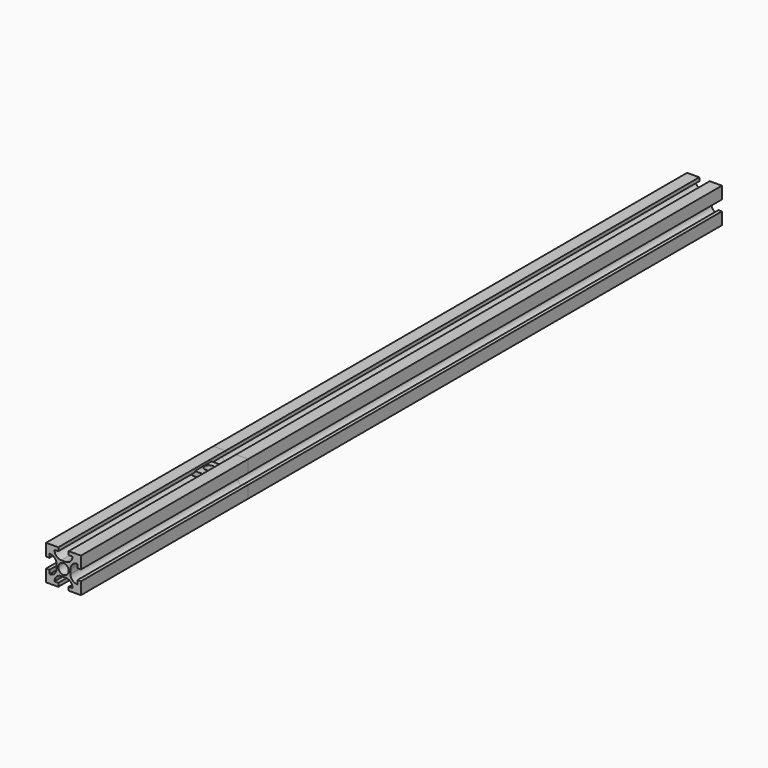
from build123d import *

# Parameters (mm, degrees)
F0_R      = 3
F1_DEPTH  = 350
F2_DEPTH  = 260
F3_DEPTH  = 460
F4_DEPTH  = 280
F5_DEPTH  = 210
F6_R      = 3
F7_DEPTH  = 20.001
F8_DEPTH  = 250
F10_DEPTH = 12
F11_R     = 2.5
F12_DEPTH = 18.701799197
F13_DEPTH = 460
F14_DEPTH = 227
F15_DEPTH = 340


with BuildPart() as f1:
    # F0 (on Front) → F1 (new body)
    with BuildSketch(Plane.XZ):
        with BuildLine():
            Line((3, 10), (3, 8))
            Line((3, 8), (5.1872519999, 8))
            ThreePointArc((5.1872519999, 8), (4.0330427178, 5.1732112188), (1.2140873587, 4))
            Line((1.2140873587, 4), (0, 4))
            Line((0, 4), (-1.2140873587, 4))
            ThreePointArc((-1.2140873587, 4), (-4.0330427178, 5.1732112188), (-5.1872519999, 8))
            Line((-5.1872519999, 8), (-3, 8))
            Line((-3, 8), (-3, 10))
            Line((-3, 10), (-10, 10))
            Line((-10, 10), (-10, 3))
            Line((-10, 3), (-8, 3))
            Line((-8, 3), (-8, 5.1872519999))
            ThreePointArc((-8, 5.1872519999), (-5.1732112188, 4.0330427178), (-4, 1.2140873587))
            Line((-4, 1.2140873587), (-4, 0))
            Line((-4, 0), (-4, -1.2140873587))
            ThreePointArc((-4, -1.2140873587), (-5.1732112188, -4.0330427178), (-8, -5.1872519999))
            Line((-8, -5.1872519999), (-8, -3))
            Line((-8, -3), (-10, -3))
            Line((-10, -3), (-10, -10))
            Line((-10, -10), (-3, -10))
            Line((-3, -10), (-3, -8))
            Line((-3, -8), (-5.1872519999, -8))
            ThreePointArc((-5.1872519999, -8), (-4.0330427178, -5.1732112188), (-1.2140873587, -4))
            Line((-1.2140873587, -4), (0, -4))
            Line((0, -4), (1.2140873587, -4))
            ThreePointArc((1.2140873587, -4), (4.0330427178, -5.1732112188), (5.1872519999, -8))
            Line((5.1872519999, -8), (3, -8))
            Line((3, -8), (3, -10))
            Line((3, -10), (10, -10))
            Line((10, -10), (10, -3))
            Line((10, -3), (8, -3))
            Line((8, -3), (8, -5.1872519999))
            ThreePointArc((8, -5.1872519999), (5.1732112188, -4.0330427178), (4, -1.2140873587))
            Line((4, -1.2140873587), (4, 0))
            Line((4, 0), (4, 1.2140873587))
            ThreePointArc((4, 1.2140873587), (5.1732112188, 4.0330427178), (8, 5.1872519999))
            Line((8, 5.1872519999), (8, 3))
            Line((8, 3), (10, 3))
            Line((10, 3), (10, 10))
            Line((10, 10), (3, 10))
        make_face()
        Circle(F0_R, mode=Mode.SUBTRACT)
    extrude(amount=F1_DEPTH)


with BuildPart() as f2:
    # F0 (on Front) → F2 (new body)
    with BuildSketch(Plane.XZ):
        with BuildLine():
            Line((3, 10), (3, 8))
            Line((3, 8), (5.1872519999, 8))
            ThreePointArc((5.1872519999, 8), (4.0330427178, 5.1732112188), (1.2140873587, 4))
            Line((1.2140873587, 4), (0, 4))
            Line((0, 4), (-1.2140873587, 4))
            ThreePointArc((-1.2140873587, 4), (-4.0330427178, 5.1732112188), (-5.1872519999, 8))
            Line((-5.1872519999, 8), (-3, 8))
            Line((-3, 8), (-3, 10))
            Line((-3, 10), (-10, 10))
            Line((-10, 10), (-10, 3))
            Line((-10, 3), (-8, 3))
            Line((-8, 3), (-8, 5.1872519999))
            ThreePointArc((-8, 5.1872519999), (-5.1732112188, 4.0330427178), (-4, 1.2140873587))
            Line((-4, 1.2140873587), (-4, 0))
            Line((-4, 0), (-4, -1.2140873587))
            ThreePointArc((-4, -1.2140873587), (-5.1732112188, -4.0330427178), (-8, -5.1872519999))
            Line((-8, -5.1872519999), (-8, -3))
            Line((-8, -3), (-10, -3))
            Line((-10, -3), (-10, -10))
            Line((-10, -10), (-3, -10))
            Line((-3, -10), (-3, -8))
            Line((-3, -8), (-5.1872519999, -8))
            ThreePointArc((-5.1872519999, -8), (-4.0330427178, -5.1732112188), (-1.2140873587, -4))
            Line((-1.2140873587, -4), (0, -4))
            Line((0, -4), (1.2140873587, -4))
            ThreePointArc((1.2140873587, -4), (4.0330427178, -5.1732112188), (5.1872519999, -8))
            Line((5.1872519999, -8), (3, -8))
            Line((3, -8), (3, -10))
            Line((3, -10), (10, -10))
            Line((10, -10), (10, -3))
            Line((10, -3), (8, -3))
            Line((8, -3), (8, -5.1872519999))
            ThreePointArc((8, -5.1872519999), (5.1732112188, -4.0330427178), (4, -1.2140873587))
            Line((4, -1.2140873587), (4, 0))
            Line((4, 0), (4, 1.2140873587))
            ThreePointArc((4, 1.2140873587), (5.1732112188, 4.0330427178), (8, 5.1872519999))
            Line((8, 5.1872519999), (8, 3))
            Line((8, 3), (10, 3))
            Line((10, 3), (10, 10))
            Line((10, 10), (3, 10))
        make_face()
        Circle(F0_R, mode=Mode.SUBTRACT)
    extrude(amount=F2_DEPTH)


with BuildPart() as f3:
    # F0 (on Front) → F3 (new body)
    with BuildSketch(Plane.XZ):
        with BuildLine():
            Line((3, 10), (3, 8))
            Line((3, 8), (5.1872519999, 8))
            ThreePointArc((5.1872519999, 8), (4.0330427178, 5.1732112188), (1.2140873587, 4))
            Line((1.2140873587, 4), (0, 4))
            Line((0, 4), (-1.2140873587, 4))
            ThreePointArc((-1.2140873587, 4), (-4.0330427178, 5.1732112188), (-5.1872519999, 8))
            Line((-5.1872519999, 8), (-3, 8))
            Line((-3, 8), (-3, 10))
            Line((-3, 10), (-10, 10))
            Line((-10, 10), (-10, 3))
            Line((-10, 3), (-8, 3))
            Line((-8, 3), (-8, 5.1872519999))
            ThreePointArc((-8, 5.1872519999), (-5.1732112188, 4.0330427178), (-4, 1.2140873587))
            Line((-4, 1.2140873587), (-4, 0))
            Line((-4, 0), (-4, -1.2140873587))
            ThreePointArc((-4, -1.2140873587), (-5.1732112188, -4.0330427178), (-8, -5.1872519999))
            Line((-8, -5.1872519999), (-8, -3))
            Line((-8, -3), (-10, -3))
            Line((-10, -3), (-10, -10))
            Line((-10, -10), (-3, -10))
            Line((-3, -10), (-3, -8))
            Line((-3, -8), (-5.1872519999, -8))
            ThreePointArc((-5.1872519999, -8), (-4.0330427178, -5.1732112188), (-1.2140873587, -4))
            Line((-1.2140873587, -4), (0, -4))
            Line((0, -4), (1.2140873587, -4))
            ThreePointArc((1.2140873587, -4), (4.0330427178, -5.1732112188), (5.1872519999, -8))
            Line((5.1872519999, -8), (3, -8))
            Line((3, -8), (3, -10))
            Line((3, -10), (10, -10))
            Line((10, -10), (10, -3))
            Line((10, -3), (8, -3))
            Line((8, -3), (8, -5.1872519999))
            ThreePointArc((8, -5.1872519999), (5.1732112188, -4.0330427178), (4, -1.2140873587))
            Line((4, -1.2140873587), (4, 0))
            Line((4, 0), (4, 1.2140873587))
            ThreePointArc((4, 1.2140873587), (5.1732112188, 4.0330427178), (8, 5.1872519999))
            Line((8, 5.1872519999), (8, 3))
            Line((8, 3), (10, 3))
            Line((10, 3), (10, 10))
            Line((10, 10), (3, 10))
        make_face()
        Circle(F0_R, mode=Mode.SUBTRACT)
    extrude(amount=F3_DEPTH)


with BuildPart() as f4:
    # F0 (on Front) → F4 (new body)
    with BuildSketch(Plane.XZ):
        with BuildLine():
            Line((3, 10), (3, 8))
            Line((3, 8), (5.1872519999, 8))
            ThreePointArc((5.1872519999, 8), (4.0330427178, 5.1732112188), (1.2140873587, 4))
            Line((1.2140873587, 4), (0, 4))
            Line((0, 4), (-1.2140873587, 4))
            ThreePointArc((-1.2140873587, 4), (-4.0330427178, 5.1732112188), (-5.1872519999, 8))
            Line((-5.1872519999, 8), (-3, 8))
            Line((-3, 8), (-3, 10))
            Line((-3, 10), (-10, 10))
            Line((-10, 10), (-10, 3))
            Line((-10, 3), (-8, 3))
            Line((-8, 3), (-8, 5.1872519999))
            ThreePointArc((-8, 5.1872519999), (-5.1732112188, 4.0330427178), (-4, 1.2140873587))
            Line((-4, 1.2140873587), (-4, 0))
            Line((-4, 0), (-4, -1.2140873587))
            ThreePointArc((-4, -1.2140873587), (-5.1732112188, -4.0330427178), (-8, -5.1872519999))
            Line((-8, -5.1872519999), (-8, -3))
            Line((-8, -3), (-10, -3))
            Line((-10, -3), (-10, -10))
            Line((-10, -10), (-3, -10))
            Line((-3, -10), (-3, -8))
            Line((-3, -8), (-5.1872519999, -8))
            ThreePointArc((-5.1872519999, -8), (-4.0330427178, -5.1732112188), (-1.2140873587, -4))
            Line((-1.2140873587, -4), (0, -4))
            Line((0, -4), (1.2140873587, -4))
            ThreePointArc((1.2140873587, -4), (4.0330427178, -5.1732112188), (5.1872519999, -8))
            Line((5.1872519999, -8), (3, -8))
            Line((3, -8), (3, -10))
            Line((3, -10), (10, -10))
            Line((10, -10), (10, -3))
            Line((10, -3), (8, -3))
            Line((8, -3), (8, -5.1872519999))
            ThreePointArc((8, -5.1872519999), (5.1732112188, -4.0330427178), (4, -1.2140873587))
            Line((4, -1.2140873587), (4, 0))
            Line((4, 0), (4, 1.2140873587))
            ThreePointArc((4, 1.2140873587), (5.1732112188, 4.0330427178), (8, 5.1872519999))
            Line((8, 5.1872519999), (8, 3))
            Line((8, 3), (10, 3))
            Line((10, 3), (10, 10))
            Line((10, 10), (3, 10))
        make_face()
        Circle(F0_R, mode=Mode.SUBTRACT)
    extrude(amount=F4_DEPTH)


with BuildPart() as f5:
    # F0 (on Front) → F5 (new body)
    with BuildSketch(Plane.XZ):
        with BuildLine():
            Line((3, 10), (3, 8))
            Line((3, 8), (5.1872519999, 8))
            ThreePointArc((5.1872519999, 8), (4.0330427178, 5.1732112188), (1.2140873587, 4))
            Line((1.2140873587, 4), (0, 4))
            Line((0, 4), (-1.2140873587, 4))
            ThreePointArc((-1.2140873587, 4), (-4.0330427178, 5.1732112188), (-5.1872519999, 8))
            Line((-5.1872519999, 8), (-3, 8))
            Line((-3, 8), (-3, 10))
            Line((-3, 10), (-10, 10))
            Line((-10, 10), (-10, 3))
            Line((-10, 3), (-8, 3))
            Line((-8, 3), (-8, 5.1872519999))
            ThreePointArc((-8, 5.1872519999), (-5.1732112188, 4.0330427178), (-4, 1.2140873587))
            Line((-4, 1.2140873587), (-4, 0))
            Line((-4, 0), (-4, -1.2140873587))
            ThreePointArc((-4, -1.2140873587), (-5.1732112188, -4.0330427178), (-8, -5.1872519999))
            Line((-8, -5.1872519999), (-8, -3))
            Line((-8, -3), (-10, -3))
            Line((-10, -3), (-10, -10))
            Line((-10, -10), (-3, -10))
            Line((-3, -10), (-3, -8))
            Line((-3, -8), (-5.1872519999, -8))
            ThreePointArc((-5.1872519999, -8), (-4.0330427178, -5.1732112188), (-1.2140873587, -4))
            Line((-1.2140873587, -4), (0, -4))
            Line((0, -4), (1.2140873587, -4))
            ThreePointArc((1.2140873587, -4), (4.0330427178, -5.1732112188), (5.1872519999, -8))
            Line((5.1872519999, -8), (3, -8))
            Line((3, -8), (3, -10))
            Line((3, -10), (10, -10))
            Line((10, -10), (10, -3))
            Line((10, -3), (8, -3))
            Line((8, -3), (8, -5.1872519999))
            ThreePointArc((8, -5.1872519999), (5.1732112188, -4.0330427178), (4, -1.2140873587))
            Line((4, -1.2140873587), (4, 0))
            Line((4, 0), (4, 1.2140873587))
            ThreePointArc((4, 1.2140873587), (5.1732112188, 4.0330427178), (8, 5.1872519999))
            Line((8, 5.1872519999), (8, 3))
            Line((8, 3), (10, 3))
            Line((10, 3), (10, 10))
            Line((10, 10), (3, 10))
        make_face()
        Circle(F0_R, mode=Mode.SUBTRACT)
    extrude(amount=F5_DEPTH)

    # F6 (on face) → F7 (cut, through all)
    with BuildSketch(Plane.XY.offset(10)):
        with Locations((0, -85)):
            Circle(F6_R)
        with Locations((0, -125)):
            Circle(F6_R)
    extrude(amount=-F7_DEPTH, mode=Mode.SUBTRACT)


with BuildPart() as f8:
    # F0 (on Front) → F8 (new body)
    with BuildSketch(Plane.XZ):
        with BuildLine():
            Line((3, 10), (3, 8))
            Line((3, 8), (5.1872519999, 8))
            ThreePointArc((5.1872519999, 8), (4.0330427178, 5.1732112188), (1.2140873587, 4))
            Line((1.2140873587, 4), (0, 4))
            Line((0, 4), (-1.2140873587, 4))
            ThreePointArc((-1.2140873587, 4), (-4.0330427178, 5.1732112188), (-5.1872519999, 8))
            Line((-5.1872519999, 8), (-3, 8))
            Line((-3, 8), (-3, 10))
            Line((-3, 10), (-10, 10))
            Line((-10, 10), (-10, 3))
            Line((-10, 3), (-8, 3))
            Line((-8, 3), (-8, 5.1872519999))
            ThreePointArc((-8, 5.1872519999), (-5.1732112188, 4.0330427178), (-4, 1.2140873587))
            Line((-4, 1.2140873587), (-4, 0))
            Line((-4, 0), (-4, -1.2140873587))
            ThreePointArc((-4, -1.2140873587), (-5.1732112188, -4.0330427178), (-8, -5.1872519999))
            Line((-8, -5.1872519999), (-8, -3))
            Line((-8, -3), (-10, -3))
            Line((-10, -3), (-10, -10))
            Line((-10, -10), (-3, -10))
            Line((-3, -10), (-3, -8))
            Line((-3, -8), (-5.1872519999, -8))
            ThreePointArc((-5.1872519999, -8), (-4.0330427178, -5.1732112188), (-1.2140873587, -4))
            Line((-1.2140873587, -4), (0, -4))
            Line((0, -4), (1.2140873587, -4))
            ThreePointArc((1.2140873587, -4), (4.0330427178, -5.1732112188), (5.1872519999, -8))
            Line((5.1872519999, -8), (3, -8))
            Line((3, -8), (3, -10))
            Line((3, -10), (10, -10))
            Line((10, -10), (10, -3))
            Line((10, -3), (8, -3))
            Line((8, -3), (8, -5.1872519999))
            ThreePointArc((8, -5.1872519999), (5.1732112188, -4.0330427178), (4, -1.2140873587))
            Line((4, -1.2140873587), (4, 0))
            Line((4, 0), (4, 1.2140873587))
            ThreePointArc((4, 1.2140873587), (5.1732112188, 4.0330427178), (8, 5.1872519999))
            Line((8, 5.1872519999), (8, 3))
            Line((8, 3), (10, 3))
            Line((10, 3), (10, 10))
            Line((10, 10), (3, 10))
        make_face()
        Circle(F0_R, mode=Mode.SUBTRACT)
    extrude(amount=F8_DEPTH)


with BuildPart() as f10:
    # F9 (on face) → F10 (new body)
    with BuildSketch(Plane.XZ.offset(350)):
        with BuildLine():
            Line((3, 8.700799197), (0, 8.700799197))
            Line((0, 8.700799197), (-3, 8.700799197))
            Line((-3, 8.700799197), (-3, 8))
            Line((-3, 8), (-5.1872519999, 8))
            ThreePointArc((-5.1872519999, 8), (-5.0533025896, 6.9499370195), (-4.646838141, 5.972511135))
            Line((-4.646838141, 5.972511135), (0, 5.972511135))
            Line((0, 5.972511135), (4.646838141, 5.972511135))
            ThreePointArc((4.646838141, 5.972511135), (5.0533025896, 6.9499370195), (5.1872519999, 8))
            Line((5.1872519999, 8), (3, 8))
            Line((3, 8), (3, 8.700799197))
        make_face()
    extrude(amount=F10_DEPTH)

    # F11 (on face) → F12 (cut, through all)
    with BuildSketch(Plane.XY.offset(8.700799197)):
        with Locations((0, -355.6039333344)):
            Circle(F11_R)
    extrude(amount=-F12_DEPTH, mode=Mode.SUBTRACT)


with BuildPart() as f13:
    # F0 (on Front) → F13 (new body)
    with BuildSketch(Plane.XZ):
        with BuildLine():
            Line((3, 10), (3, 8))
            Line((3, 8), (5.1872519999, 8))
            ThreePointArc((5.1872519999, 8), (4.0330427178, 5.1732112188), (1.2140873587, 4))
            Line((1.2140873587, 4), (0, 4))
            Line((0, 4), (-1.2140873587, 4))
            ThreePointArc((-1.2140873587, 4), (-4.0330427178, 5.1732112188), (-5.1872519999, 8))
            Line((-5.1872519999, 8), (-3, 8))
            Line((-3, 8), (-3, 10))
            Line((-3, 10), (-10, 10))
            Line((-10, 10), (-10, 3))
            Line((-10, 3), (-8, 3))
            Line((-8, 3), (-8, 5.1872519999))
            ThreePointArc((-8, 5.1872519999), (-5.1732112188, 4.0330427178), (-4, 1.2140873587))
            Line((-4, 1.2140873587), (-4, 0))
            Line((-4, 0), (-4, -1.2140873587))
            ThreePointArc((-4, -1.2140873587), (-5.1732112188, -4.0330427178), (-8, -5.1872519999))
            Line((-8, -5.1872519999), (-8, -3))
            Line((-8, -3), (-10, -3))
            Line((-10, -3), (-10, -10))
            Line((-10, -10), (-3, -10))
            Line((-3, -10), (-3, -8))
            Line((-3, -8), (-5.1872519999, -8))
            ThreePointArc((-5.1872519999, -8), (-4.0330427178, -5.1732112188), (-1.2140873587, -4))
            Line((-1.2140873587, -4), (0, -4))
            Line((0, -4), (1.2140873587, -4))
            ThreePointArc((1.2140873587, -4), (4.0330427178, -5.1732112188), (5.1872519999, -8))
            Line((5.1872519999, -8), (3, -8))
            Line((3, -8), (3, -10))
            Line((3, -10), (10, -10))
            Line((10, -10), (10, -3))
            Line((10, -3), (8, -3))
            Line((8, -3), (8, -5.1872519999))
            ThreePointArc((8, -5.1872519999), (5.1732112188, -4.0330427178), (4, -1.2140873587))
            Line((4, -1.2140873587), (4, 0))
            Line((4, 0), (4, 1.2140873587))
            ThreePointArc((4, 1.2140873587), (5.1732112188, 4.0330427178), (8, 5.1872519999))
            Line((8, 5.1872519999), (8, 3))
            Line((8, 3), (10, 3))
            Line((10, 3), (10, 10))
            Line((10, 10), (3, 10))
        make_face()
        Circle(F0_R, mode=Mode.SUBTRACT)
    extrude(amount=F13_DEPTH)


with BuildPart() as f14:
    # F0 (on Front) → F14 (new body)
    with BuildSketch(Plane.XZ):
        with BuildLine():
            Line((3, 10), (3, 8))
            Line((3, 8), (5.1872519999, 8))
            ThreePointArc((5.1872519999, 8), (4.0330427178, 5.1732112188), (1.2140873587, 4))
            Line((1.2140873587, 4), (0, 4))
            Line((0, 4), (-1.2140873587, 4))
            ThreePointArc((-1.2140873587, 4), (-4.0330427178, 5.1732112188), (-5.1872519999, 8))
            Line((-5.1872519999, 8), (-3, 8))
            Line((-3, 8), (-3, 10))
            Line((-3, 10), (-10, 10))
            Line((-10, 10), (-10, 3))
            Line((-10, 3), (-8, 3))
            Line((-8, 3), (-8, 5.1872519999))
            ThreePointArc((-8, 5.1872519999), (-5.1732112188, 4.0330427178), (-4, 1.2140873587))
            Line((-4, 1.2140873587), (-4, 0))
            Line((-4, 0), (-4, -1.2140873587))
            ThreePointArc((-4, -1.2140873587), (-5.1732112188, -4.0330427178), (-8, -5.1872519999))
            Line((-8, -5.1872519999), (-8, -3))
            Line((-8, -3), (-10, -3))
            Line((-10, -3), (-10, -10))
            Line((-10, -10), (-3, -10))
            Line((-3, -10), (-3, -8))
            Line((-3, -8), (-5.1872519999, -8))
            ThreePointArc((-5.1872519999, -8), (-4.0330427178, -5.1732112188), (-1.2140873587, -4))
            Line((-1.2140873587, -4), (0, -4))
            Line((0, -4), (1.2140873587, -4))
            ThreePointArc((1.2140873587, -4), (4.0330427178, -5.1732112188), (5.1872519999, -8))
            Line((5.1872519999, -8), (3, -8))
            Line((3, -8), (3, -10))
            Line((3, -10), (10, -10))
            Line((10, -10), (10, -3))
            Line((10, -3), (8, -3))
            Line((8, -3), (8, -5.1872519999))
            ThreePointArc((8, -5.1872519999), (5.1732112188, -4.0330427178), (4, -1.2140873587))
            Line((4, -1.2140873587), (4, 0))
            Line((4, 0), (4, 1.2140873587))
            ThreePointArc((4, 1.2140873587), (5.1732112188, 4.0330427178), (8, 5.1872519999))
            Line((8, 5.1872519999), (8, 3))
            Line((8, 3), (10, 3))
            Line((10, 3), (10, 10))
            Line((10, 10), (3, 10))
        make_face()
        Circle(F0_R, mode=Mode.SUBTRACT)
    extrude(amount=F14_DEPTH)


with BuildPart() as f15:
    # F0 (on Front) → F15 (new body)
    with BuildSketch(Plane.XZ):
        with BuildLine():
            Line((3, 10), (3, 8))
            Line((3, 8), (5.1872519999, 8))
            ThreePointArc((5.1872519999, 8), (4.0330427178, 5.1732112188), (1.2140873587, 4))
            Line((1.2140873587, 4), (0, 4))
            Line((0, 4), (-1.2140873587, 4))
            ThreePointArc((-1.2140873587, 4), (-4.0330427178, 5.1732112188), (-5.1872519999, 8))
            Line((-5.1872519999, 8), (-3, 8))
            Line((-3, 8), (-3, 10))
            Line((-3, 10), (-10, 10))
            Line((-10, 10), (-10, 3))
            Line((-10, 3), (-8, 3))
            Line((-8, 3), (-8, 5.1872519999))
            ThreePointArc((-8, 5.1872519999), (-5.1732112188, 4.0330427178), (-4, 1.2140873587))
            Line((-4, 1.2140873587), (-4, 0))
            Line((-4, 0), (-4, -1.2140873587))
            ThreePointArc((-4, -1.2140873587), (-5.1732112188, -4.0330427178), (-8, -5.1872519999))
            Line((-8, -5.1872519999), (-8, -3))
            Line((-8, -3), (-10, -3))
            Line((-10, -3), (-10, -10))
            Line((-10, -10), (-3, -10))
            Line((-3, -10), (-3, -8))
            Line((-3, -8), (-5.1872519999, -8))
            ThreePointArc((-5.1872519999, -8), (-4.0330427178, -5.1732112188), (-1.2140873587, -4))
            Line((-1.2140873587, -4), (0, -4))
            Line((0, -4), (1.2140873587, -4))
            ThreePointArc((1.2140873587, -4), (4.0330427178, -5.1732112188), (5.1872519999, -8))
            Line((5.1872519999, -8), (3, -8))
            Line((3, -8), (3, -10))
            Line((3, -10), (10, -10))
            Line((10, -10), (10, -3))
            Line((10, -3), (8, -3))
            Line((8, -3), (8, -5.1872519999))
            ThreePointArc((8, -5.1872519999), (5.1732112188, -4.0330427178), (4, -1.2140873587))
            Line((4, -1.2140873587), (4, 0))
            Line((4, 0), (4, 1.2140873587))
            ThreePointArc((4, 1.2140873587), (5.1732112188, 4.0330427178), (8, 5.1872519999))
            Line((8, 5.1872519999), (8, 3))
            Line((8, 3), (10, 3))
            Line((10, 3), (10, 10))
            Line((10, 10), (3, 10))
        make_face()
        Circle(F0_R, mode=Mode.SUBTRACT)
    extrude(amount=F15_DEPTH)


solid = Compound([f1.part, f2.part, f3.part, f4.part, f5.part, f8.part, f10.part, f13.part, f14.part, f15.part])
